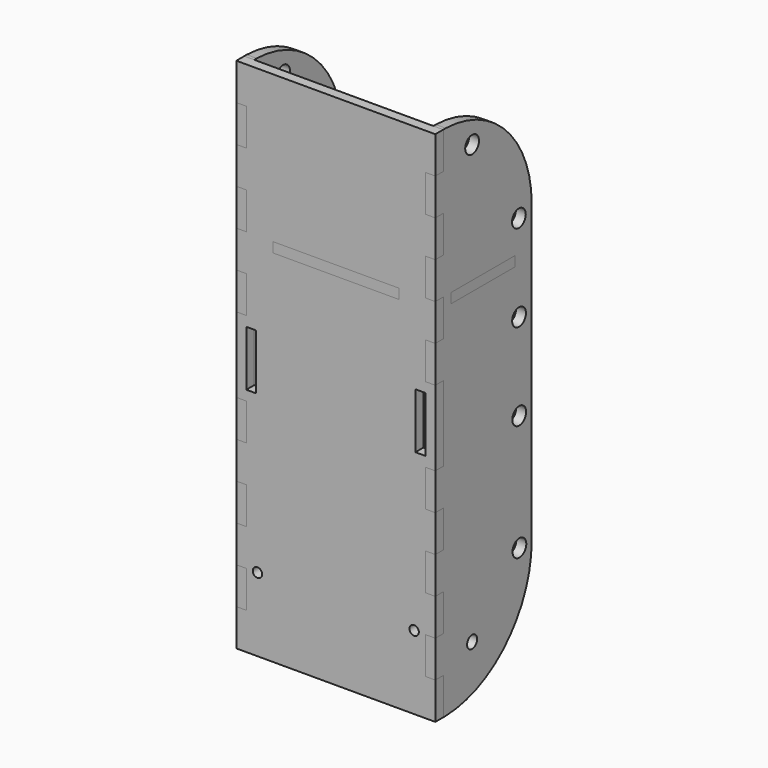
from build123d import *

# Parameters (mm, degrees)
F3_R      = 1.5
F3_W      = 3.175
F3_H      = 17.69
F4_DEPTH  = 3.175
F6_START  = 28.575
F5_R      = 2
F5_R_2    = 2.75
F6_DEPTH  = 3.175
F9_START  = 91.395
F9_DEPTH  = 3.175
F10_START = 91.395
F10_DEPTH = 3.175


# Not quite as in the source:
# - a variable given as a bare number and used for a length is read in inches; the dataset says mm whatever the document's units were


with BuildPart() as f4:
    # F3 (on Front) → F4 (new body)
    with BuildSketch(Plane.XZ):
        Polygon((-31.75, -23.51), (0, -23.51), (31.75, -23.51), (31.75, -11.755), (28.575, -11.755), (28.575, 0), (31.75, 0), (31.75, 11.755), (28.575, 11.755), (28.575, 23.51), (31.75, 23.51), (31.75, 35.265), (28.575, 35.265), (28.575, 47.02), (31.75, 47.02), (31.75, 59.04), (31.75, 71.06), (28.575, 71.06), (28.575, 82.815), (31.75, 82.815), (31.75, 94.57), (28.575, 94.57), (28.575, 106.325), (31.75, 106.325), (31.75, 118.08), (28.575, 118.08), (28.575, 129.835), (31.75, 129.835), (31.75, 141.59), (0, 141.59), (-31.75, 141.59), (-31.75, 129.835), (-28.575, 129.835), (-28.575, 118.08), (-31.75, 118.08), (-31.75, 106.325), (-28.575, 106.325), (-28.575, 94.57), (-31.75, 94.57), (-31.75, 82.815), (-28.575, 82.815), (-28.575, 71.06), (-31.75, 71.06), (-31.75, 59.04), (-31.75, 47.02), (-28.575, 47.02), (-28.575, 35.265), (-31.75, 35.265), (-31.75, 23.51), (-28.575, 23.51), (-28.575, 11.755), (-31.75, 11.755), (-31.75, 0), (-28.575, 0), (-28.575, -11.755), (-31.75, -11.755), align=None)
        with Locations((-25, 0)):
            Circle(F3_R, mode=Mode.SUBTRACT)
        with Locations((-26.9875, 59.04)):
            Rectangle(F3_W, F3_H, mode=Mode.SUBTRACT)
        with Locations((25, 0)):
            Circle(F3_R, mode=Mode.SUBTRACT)
        with Locations((26.9875, 59.04)):
            Rectangle(F3_W, F3_H, mode=Mode.SUBTRACT)
    extrude(amount=F4_DEPTH)


with BuildPart() as f6:
    # F5 (on Right) → F6 (new body)
    with BuildSketch(Plane.YZ.offset(F6_START)):
        with BuildLine():
            Line((0, -11.755), (0, -23.51))
            Line((0, -23.51), (0.9683232056, -23.51))
            ThreePointArc((0.9683232056, -23.51), (25.2855557925, -12.8457833838), (35.2782918355, 11.755))
            Line((35.2782918355, 11.755), (35.2782918355, 106.325))
            ThreePointArc((35.2782918355, 106.325), (25.2855557925, 130.9257833838), (0.9683232056, 141.59))
            Line((0.9683232056, 141.59), (0, 141.59))
            Line((0, 141.59), (0, 129.835))
            Line((0, 129.835), (-3.175, 129.835))
            Line((-3.175, 129.835), (-3.175, 118.08))
            Line((-3.175, 118.08), (0, 118.08))
            Line((0, 118.08), (0, 106.325))
            Line((0, 106.325), (-3.175, 106.325))
            Line((-3.175, 106.325), (-3.175, 94.57))
            Line((-3.175, 94.57), (0, 94.57))
            Line((0, 94.57), (0, 82.815))
            Line((0, 82.815), (-3.175, 82.815))
            Line((-3.175, 82.815), (-3.175, 71.06))
            Line((-3.175, 71.06), (0, 71.06))
            Line((0, 71.06), (0, 59.04))
            Line((0, 59.04), (0, 47.02))
            Line((0, 47.02), (-3.175, 47.02))
            Line((-3.175, 47.02), (-3.175, 35.265))
            Line((-3.175, 35.265), (0, 35.265))
            Line((0, 35.265), (0, 23.51))
            Line((0, 23.51), (-3.175, 23.51))
            Line((-3.175, 23.51), (-3.175, 11.755))
            Line((-3.175, 11.755), (0, 11.755))
            Line((0, 11.755), (0, 0))
            Line((0, 0), (-3.175, 0))
            Line((-3.175, 0), (-3.175, -11.755))
            Line((-3.175, -11.755), (0, -11.755))
        make_face()
        with Locations((11.5, -7)):
            Circle(F5_R, mode=Mode.SUBTRACT)
        with Locations((30.370771822, 11.755)):
            Circle(F5_R_2, mode=Mode.SUBTRACT)
        with Locations((30.3006969122, 48.8940113736)):
            Circle(F5_R_2, mode=Mode.SUBTRACT)
        with Locations((11.5, 132.7)):
            Circle(F5_R_2, mode=Mode.SUBTRACT)
        with Locations((30.2306220023, 76.6660547871)):
            Circle(F5_R_2, mode=Mode.SUBTRACT)
        with Locations((30.1605470924, 104.4380982005)):
            Circle(F5_R_2, mode=Mode.SUBTRACT)
    extrude(amount=F6_DEPTH)


with BuildPart() as f7_1:
    # F7: instance of F6
    add(f6.part.mirror(Plane.YZ))


with BuildPart() as f9_tool:
    # F8 (on Top) → F9 (new body)
    with BuildSketch(Plane.XY.offset(F9_START)):
        Polygon((20.1083333333, 11.5), (0, 11.5), (-20.1083333333, 11.5), (-28.575, 31.75), (-28.575, 28.575), (-31.75, 28.575), (-31.75, 3.175), (-28.575, 3.175), (-28.575, 0), (-20.1083333333, 0), (-20.1083333333, -3.175), (0, -3.175), (20.1083333333, -3.175), (20.1083333333, 0), (28.575, 0), (28.575, 3.175), (31.75, 3.175), (31.75, 28.575), (28.575, 28.575), (28.575, 31.75), align=None)
    extrude(amount=F9_DEPTH)


with BuildPart() as f4_1:
    add(f4.part)

    # F9: cut by f9_tool
    add(f9_tool.part, mode=Mode.SUBTRACT)


with BuildPart() as f6_1:
    add(f6.part)

    # F9: cut by f9_tool
    add(f9_tool.part, mode=Mode.SUBTRACT)


with BuildPart() as f7_1_1:
    add(f7_1.part)

    # F9: cut by f9_tool
    add(f9_tool.part, mode=Mode.SUBTRACT)


with BuildPart() as f10:
    # F8 (on Top) → F10 (new body)
    with BuildSketch(Plane.XY.offset(F10_START)):
        Polygon((20.1083333333, 11.5), (0, 11.5), (-20.1083333333, 11.5), (-28.575, 31.75), (-28.575, 28.575), (-31.75, 28.575), (-31.75, 3.175), (-28.575, 3.175), (-28.575, 0), (-20.1083333333, 0), (-20.1083333333, -3.175), (0, -3.175), (20.1083333333, -3.175), (20.1083333333, 0), (28.575, 0), (28.575, 3.175), (31.75, 3.175), (31.75, 28.575), (28.575, 28.575), (28.575, 31.75), align=None)
    extrude(amount=F10_DEPTH)


solid = Compound([f4_1.part, f6_1.part, f7_1_1.part, f10.part])
